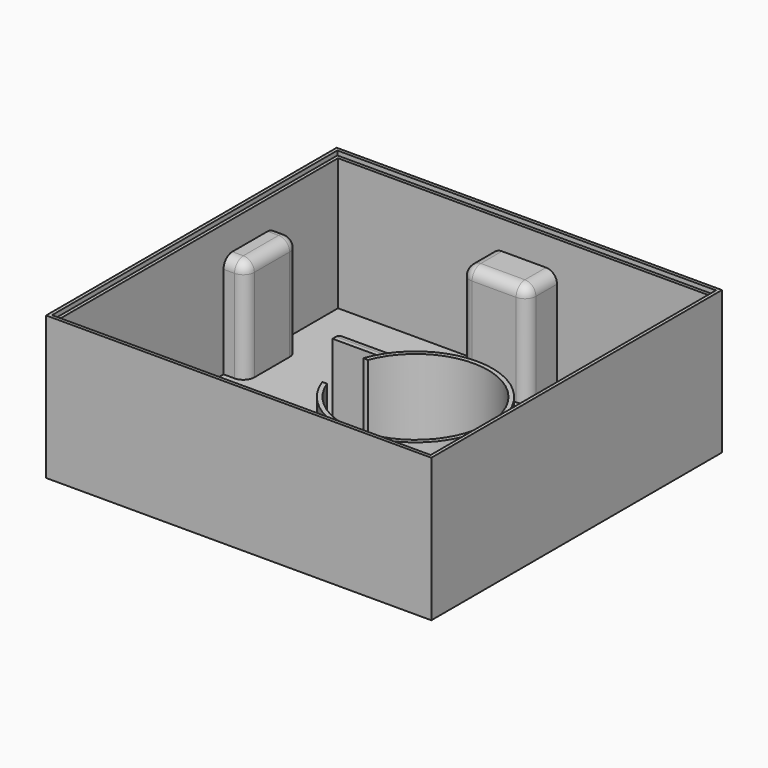
from build123d import *

# Parameters (mm, degrees)
F0_W          = 172
F0_H          = 162
F1_DEPTH      = 63
F2_DEPTH      = 3
F3_DEPTH      = 50
F4_DEPTH      = 10
F5_F1_R       = 5
F5_F2_R       = 5
F5_2_F1_R     = 5
F5_2_F2_R     = 5
F5_2_F3_R     = 5
F5_3_T1_DEPTH = 55
F5_3_T3_DEPTH = 75
F5_4_F1_R     = 5
F5_4_F2_R     = 5
F5_4_F3_R     = 5
F6_DEPTH      = 65


# Not quite as in the source:
# - a fillet or chamfer that OpenCascade refuses, or shapes differently, is made with other operations: its cross-section is extruded or revolved along the edge and cut away or added


with BuildPart() as f1:
    # F0 (on Top) → F1 (new body)
    with BuildSketch(Plane.XY):
        Polygon((-87.5, -82.5), (87.5, -82.5), (87.5, -81), (87.5, 82.5), (0, 82.5), (-87.5, 82.5), align=None)
        Rectangle(F0_W, F0_H, mode=Mode.SUBTRACT)
        Rectangle(F0_W, F0_H)
        with BuildLine():
            Line((84.5, -58.1619037897), (84.5, -79.5))
            Line((84.5, -79.5), (63.1619037897, -79.5))
            ThreePointArc((63.1619037897, -79.5), (76.2487373415, -71.2487373415), (84.5, -58.1619037897))
        make_face(mode=Mode.SUBTRACT)
        with BuildLine():
            Line((-84.5, 44.5), (-84.5, 79.5))
            Line((-84.5, 79.5), (-15, 79.5))
            Line((-15, 79.5), (15, 79.5))
            Line((15, 79.5), (84.5, 79.5))
            Line((84.5, 79.5), (84.5, 44.5))
            Line((84.5, 44.5), (84.5, 14.5))
            Line((84.5, 14.5), (84.5, -34.8380962103))
            ThreePointArc((84.5, -34.8380962103), (51.5, -11.5), (18.5, -34.8380962103))
            Line((18.5, -34.8380962103), (20.6293019191, -34.8380962103))
            ThreePointArc((20.6293019191, -34.8380962103), (84.5, -46.5), (20.6293019191, -58.1619037897))
            Line((20.6293019191, -58.1619037897), (18.5, -58.1619037897))
            ThreePointArc((18.5, -58.1619037897), (26.7512626585, -71.2487373415), (39.8380962103, -79.5))
            Line((39.8380962103, -79.5), (-84.5, -79.5))
            Line((-84.5, -79.5), (-84.5, 14.5))
            Line((-84.5, 14.5), (-84.5, 44.5))
        make_face(mode=Mode.SUBTRACT)
    extrude(amount=F1_DEPTH)


with BuildPart() as f2:
    # F0 (on Top) → F2 (new body)
    with BuildSketch(Plane.XY):
        with BuildLine():
            Line((-15, 79.5), (-84.5, 79.5))
            Line((-84.5, 79.5), (-84.5, 44.5))
            Line((-84.5, 44.5), (-74.5, 44.5))
            Line((-74.5, 44.5), (-74.5, 29.5))
            Line((-74.5, 29.5), (-74.5, 14.5))
            Line((-74.5, 14.5), (-84.5, 14.5))
            Line((-84.5, 14.5), (-84.5, -79.5))
            Line((-84.5, -79.5), (39.8380962103, -79.5))
            ThreePointArc((39.8380962103, -79.5), (26.7512626585, -71.2487373415), (18.5, -58.1619037897))
            Line((18.5, -58.1619037897), (20.6293019191, -58.1619037897))
            ThreePointArc((20.6293019191, -58.1619037897), (84.5, -46.5), (20.6293019191, -34.8380962103))
            Line((20.6293019191, -34.8380962103), (18.5, -34.8380962103))
            ThreePointArc((18.5, -34.8380962103), (51.5, -11.5), (84.5, -34.8380962103))
            Line((84.5, -34.8380962103), (84.5, 14.5))
            Line((84.5, 14.5), (65.5, 14.5))
            Line((65.5, 14.5), (55.5, 14.5))
            Line((55.5, 14.5), (55.5, 44.5))
            Line((55.5, 44.5), (65.5, 44.5))
            Line((65.5, 44.5), (84.5, 44.5))
            Line((84.5, 44.5), (84.5, 79.5))
            Line((84.5, 79.5), (15, 79.5))
            Line((15, 79.5), (15, 62.5))
            Line((15, 62.5), (0, 62.5))
            Line((0, 62.5), (-15, 62.5))
            Line((-15, 62.5), (-15, 79.5))
        make_face()
        Polygon((-15, -3.5), (0, -3.5), (15, -3.5), (15, -10.5), (-15, -10.5), align=None, mode=Mode.SUBTRACT)
        Polygon((-74.5, 44.5), (-84.5, 44.5), (-84.5, 14.5), (-74.5, 14.5), (-74.5, 29.5), align=None)
        Polygon((15, 79.5), (-15, 79.5), (-15, 62.5), (0, 62.5), (15, 62.5), align=None)
        Polygon((65.5, 29.5), (65.5, 44.5), (55.5, 44.5), (55.5, 14.5), (65.5, 14.5), align=None)
        Polygon((84.5, 14.5), (84.5, 44.5), (65.5, 44.5), (65.5, 29.5), (65.5, 14.5), align=None)
        Polygon((15, -3.5), (0, -3.5), (-15, -3.5), (-15, -10.5), (15, -10.5), align=None)
    extrude(amount=F2_DEPTH)


with BuildPart() as f2b:
    # F0 (on Top) → F2, piece 2 (new body)
    with BuildSketch(Plane.XY):
        with BuildLine():
            Line((63.1619037897, -79.5), (84.5, -79.5))
            Line((84.5, -79.5), (84.5, -58.1619037897))
            ThreePointArc((84.5, -58.1619037897), (76.2487373415, -71.2487373415), (63.1619037897, -79.5))
        make_face()
    extrude(amount=F2_DEPTH)


with BuildPart() as f3:
    # F0 (on Top) → F3 (new body)
    with BuildSketch(Plane.XY):
        Polygon((84.5, 14.5), (84.5, 44.5), (65.5, 44.5), (65.5, 29.5), (65.5, 14.5), align=None)
    extrude(amount=F3_DEPTH)

    # F0 (on Top) → F4 (join)
    with BuildSketch(Plane.XY):
        Polygon((65.5, 29.5), (65.5, 44.5), (55.5, 44.5), (55.5, 14.5), (65.5, 14.5), align=None)
    extrude(amount=F4_DEPTH)

    # F5: fillet of radius 5 on 6 edges, made by hand

    # F5_f1
    f5_f1_edges = [f3.edges().sort_by_distance(p)[0] for p in [
        (65.5, 29.5, 10),
    ]]
    fillet(f5_f1_edges, radius=F5_F1_R)

    # F5_f2
    f5_f2_edges = [f3.edges().sort_by_distance(p)[0] for p in [
        (65.5, 14.5, 32.5),
        (65.5, 29.5, 50),
        (65.5, 44.5, 32.5),
        (75, 14.5, 50),
        (75, 44.5, 50),
        (64.0355339059, 44.5, 11.4644660941),
        (64.0355339059, 14.5, 11.4644660941),
    ]]
    fillet(f5_f2_edges, radius=F5_F2_R)


with BuildPart() as f3b:
    # F0 (on Top) → F3, piece 2 (new body)
    with BuildSketch(Plane.XY):
        Polygon((15, 79.5), (-15, 79.5), (-15, 62.5), (0, 62.5), (15, 62.5), align=None)
    extrude(amount=F3_DEPTH)

    # F5#2: fillet of radius 5 on 5 edges, made by hand

    # F5_2_f1
    f5_2_f1_edges = [f3b.edges().sort_by_distance(p)[0] for p in [
        (-15, 71, 50),
    ]]
    fillet(f5_2_f1_edges, radius=F5_2_F1_R)

    # F5_2_f2
    f5_2_f2_edges = [f3b.edges().sort_by_distance(p)[0] for p in [
        (2.5, 62.5, 50),
    ]]
    fillet(f5_2_f2_edges, radius=F5_2_F2_R)

    # F5_2_f3
    f5_2_f3_edges = [f3b.edges().sort_by_distance(p)[0] for p in [
        (15, 73.5, 50),
    ]]
    fillet(f5_2_f3_edges, radius=F5_2_F3_R)


with BuildPart() as f3c:
    # F0 (on Top) → F3, piece 3 (new body)
    with BuildSketch(Plane.XY):
        Polygon((15, -3.5), (0, -3.5), (-15, -3.5), (-15, -10.5), (15, -10.5), align=None)
    extrude(amount=F3_DEPTH)

    # F5#3: fillet of radius 5 on 3 edges, made by hand

    # F5_3_s2 → F5_3_t1 (cut)
    with BuildSketch(Plane.YZ.offset(-27.5)):
        with BuildLine():
            ThreePointArc((-3.5, 45), (-4.9644660941, 48.5355339059), (-8.5, 50))
            Line((-8.5, 50), (-3.5, 50))
            Line((-3.5, 50), (-3.5, 45))
        make_face()
    extrude(amount=F5_3_T1_DEPTH, mode=Mode.SUBTRACT)

    # F5_3_s4 → F5_3_t3 (cut)
    with BuildSketch(Plane.XY.offset(-12.5)):
        with BuildLine():
            ThreePointArc((-10, -3.5), (-13.5355339059, -4.9644660941), (-15, -8.5))
            Line((-15, -8.5), (-15, -3.5))
            Line((-15, -3.5), (-10, -3.5))
        make_face()
        with BuildLine():
            ThreePointArc((10, -3.5), (13.5355339059, -4.9644660941), (15, -8.5))
            Line((15, -8.5), (15, -3.5))
            Line((15, -3.5), (10, -3.5))
        make_face()
    extrude(amount=F5_3_T3_DEPTH, mode=Mode.SUBTRACT)


with BuildPart() as f3d:
    # F0 (on Top) → F3, piece 4 (new body)
    with BuildSketch(Plane.XY):
        Polygon((-74.5, 44.5), (-84.5, 44.5), (-84.5, 14.5), (-74.5, 14.5), (-74.5, 29.5), align=None)
    extrude(amount=F3_DEPTH)

    # F5#4: fillet of radius 5 on 5 edges, made by hand

    # F5_4_f1
    f5_4_f1_edges = [f3d.edges().sort_by_distance(p)[0] for p in [
        (-74.5, 44.5, 25),
    ]]
    fillet(f5_4_f1_edges, radius=F5_4_F1_R)

    # F5_4_f2
    f5_4_f2_edges = [f3d.edges().sort_by_distance(p)[0] for p in [
        (-82, 44.5, 50),
    ]]
    fillet(f5_4_f2_edges, radius=F5_4_F2_R)

    # F5_4_f3
    f5_4_f3_edges = [f3d.edges().sort_by_distance(p)[0] for p in [
        (-82, 14.5, 50),
    ]]
    fillet(f5_4_f3_edges, radius=F5_4_F3_R)


with BuildPart() as f6:
    # F0 (on Top) → F6 (new body)
    with BuildSketch(Plane.XY):
        Polygon((-87.5, -82.5), (87.5, -82.5), (87.5, -81), (87.5, 82.5), (0, 82.5), (-87.5, 82.5), align=None)
        Rectangle(F0_W, F0_H, mode=Mode.SUBTRACT)
    extrude(amount=F6_DEPTH)


solid = Compound([f1.part, f2.part, f2b.part, f3.part, f3b.part, f3c.part, f3d.part, f6.part])
